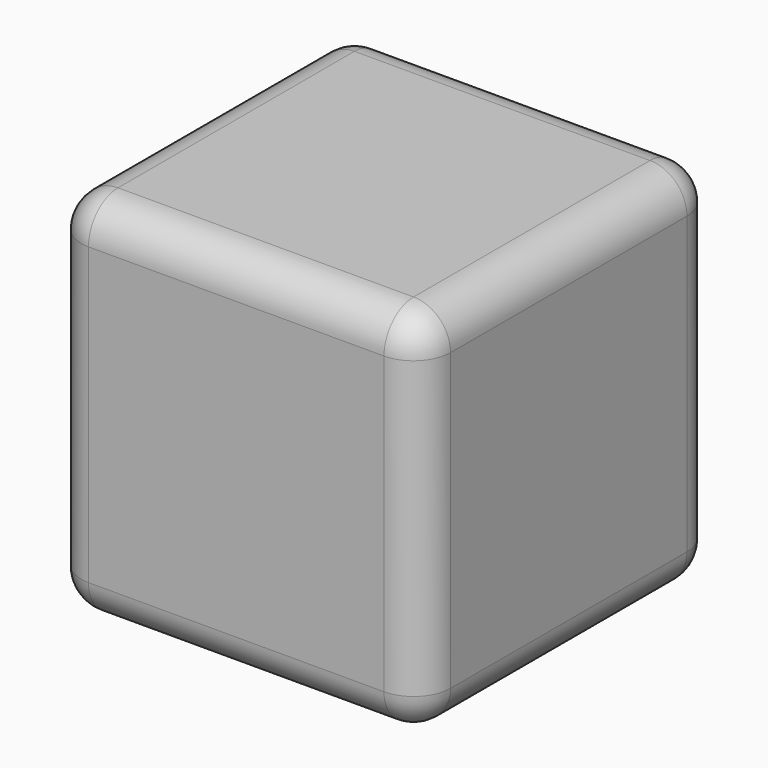
from build123d import *

# Parameters (mm, degrees)
F0_W      = 101.6
F0_H      = 101.6
F1_DEPTH  = 101.6
F2_R      = 50.8
F3_DEPTH  = 101.6
F9_W      = 101.6
F9_H      = 101.6
F10_DEPTH = 101.6
F11_R     = 10.16
F12_W     = 81.28
F12_H     = 81.28
F14_DEPTH = 88.9


# Not quite as in the source:
# - a feature of the source that left no trace in its solid (it failed there, or was rolled back) is left out


with BuildPart() as f1:
    # F0 (on Top) → F1 (new body)
    with BuildSketch(Plane.XY):
        Rectangle(F0_W, F0_H)
    extrude(amount=F1_DEPTH)


with BuildPart() as f3:
    # F2 (on Top) → F3 (new body)
    with BuildSketch(Plane.XY):
        Circle(F2_R)
    extrude(amount=F3_DEPTH)


with BuildPart() as f5:
    # F4 (on Front) → F5 (revolve)
    with BuildSketch(Plane.XZ):
        with BuildLine():
            Line((-42.8895973013, 27.2235641188), (42.8895973013, -27.2235641188))
            ThreePointArc((42.8895973013, -27.2235641188), (27.2235641188, 42.8895973013), (-42.8895973013, 27.2235641188))
        make_face()
    revolve(axis=Axis((0, 0, 0), (0.8442834114, 0, -0.5358969315)))


with BuildPart() as f10:
    # F9 (on Top) → F10 (new body)
    with BuildSketch(Plane.XY):
        Rectangle(F9_W, F9_H)
    extrude(amount=F10_DEPTH)

    # F11
    f11_edges = [f10.edges().sort_by_distance(p)[0] for p in [
        (-50.8, 50.8, 50.8),
        (-50.8, 0, 101.6),
        (0, 50.8, 101.6),
        (50.8, 0, 101.6),
        (50.8, 50.8, 50.8),
        (50.8, -50.8, 50.8),
        (50.8, 0, 0),
        (0, -50.8, 0),
        (-50.8, -50.8, 50.8),
        (-50.8, 0, 0),
        (0, 50.8, 0),
        (0, -50.8, 101.6),
    ]]
    fillet(f11_edges, radius=F11_R)

    # F12 (on face) → F14 (cut)
    with BuildSketch(Plane(origin=(0, 0, 0), x_dir=(1, 0, 0), z_dir=(0, 0, -1))):
        Rectangle(F12_W, F12_H)
    extrude(amount=-F14_DEPTH, mode=Mode.SUBTRACT)


solid = f10.part
